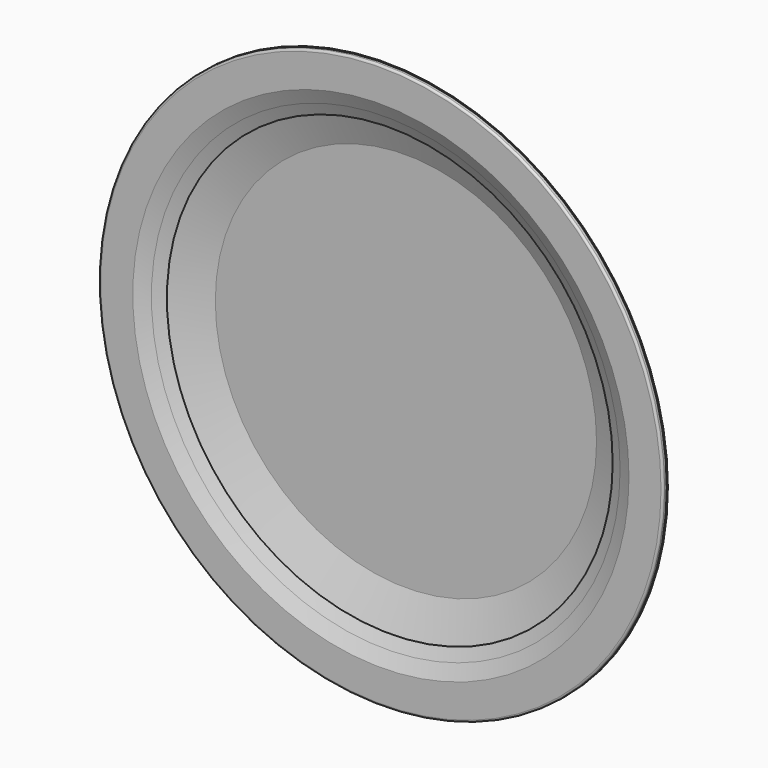
from build123d import *

# Parameters (mm, degrees)
F0_R           = 95
F1_DEPTH       = 5
F2_T           = -0.9
F4_R           = 140
F5_DEPTH       = 3
F1_FACE_R      = 95
F5_FACE_R      = 140
F8_R           = 1
F9_T           = -2.5
F10_W          = 7.818793878
F10_H          = 3.2596825622
F11_DEPTH      = 109.4
F11_DEPTH_BACK = 153.9
F12_W          = 3.6079295565
F12_H          = 7.81879
F13_DEPTH      = 116
F13_DEPTH_BACK = 123
F14_W          = 73.1657221913
F14_H          = 65.6104907393
F15_DEPTH      = 0.01


# Not quite as in the source:
# - a feature of the source that left no trace in its solid (it failed there, or was rolled back) is left out


with BuildPart() as f1:
    # F0 (on Front) → F1 (new body)
    with BuildSketch(Plane.XZ):
        Circle(F0_R)
    extrude(amount=F1_DEPTH)

    # F2
    f2_openings = [f1.faces().sort_by_distance(p)[0] for p in [
        (0, 0, 0),
    ]]
    offset(amount=F2_T, openings=f2_openings)

    # F10 (on Top) → F11 (cut, two sides)
    with BuildSketch(Plane.XY) as f11_sk:
        Rectangle(F10_W, F10_H)
    extrude(amount=-F11_DEPTH, mode=Mode.SUBTRACT)
    extrude(f11_sk.sketch, amount=F11_DEPTH_BACK, mode=Mode.SUBTRACT)

    # F12 (on Right) → F13 (cut, two sides)
    with BuildSketch(Plane.YZ) as f13_sk:
        Rectangle(F12_W, F12_H)
    extrude(amount=-F13_DEPTH, mode=Mode.SUBTRACT)
    extrude(f13_sk.sketch, amount=F13_DEPTH_BACK, mode=Mode.SUBTRACT)


with BuildPart() as f5:
    # F4 (on offset) → F5 (new body)
    with BuildSketch(Plane.XZ.offset(20)):
        Circle(F4_R)
    extrude(amount=F5_DEPTH)

    # F8
    f8_edges = [f5.edges().sort_by_distance(p)[0] for p in [
        (-140, -20, 0),
        (-140, -23, 0),
    ]]
    fillet(f8_edges, radius=F8_R)


with BuildPart() as f6:
    # F1_face (on face) → F6 section 0
    with BuildSketch(Plane.XZ.offset(5)):
        Circle(F1_FACE_R)
    # F5_face (on face) → F6 section 1
    with BuildSketch(Plane(origin=(0, -20, 0), x_dir=(1, 0, 0), z_dir=(0, 1, 0))):
        Circle(F5_FACE_R)
    loft()

    # F9 (hollow: no face is removed)
    offset(amount=F9_T, mode=Mode.SUBTRACT)


with BuildPart() as f15:
    # F14 (on Front) → F15 (new body)
    with BuildSketch(Plane.XZ):
        Rectangle(F14_W, F14_H)
    extrude(amount=F15_DEPTH)


with BuildPart() as f17_tool:
    # F16 (on Top) → F17 (revolve)
    with BuildSketch(Plane.XY):
        Polygon((93.0999964476, -9.8000001162), (0, -9.8000001162), (0, -30.2647054195), (126.5352964401, -24.4999993593), align=None)
    revolve(axis=Axis((0, -20.0323527679, 0), (0, -1, 0)))


with BuildPart() as f5_1:
    add(f5.part)

    # F17: cut by f17_tool
    add(f17_tool.part, mode=Mode.SUBTRACT)


with BuildPart() as f6_1:
    add(f6.part)

    # F17: cut by f17_tool
    add(f17_tool.part, mode=Mode.SUBTRACT)


solid = Compound([f1.part, f15.part, f5_1.part, f6_1.part])
